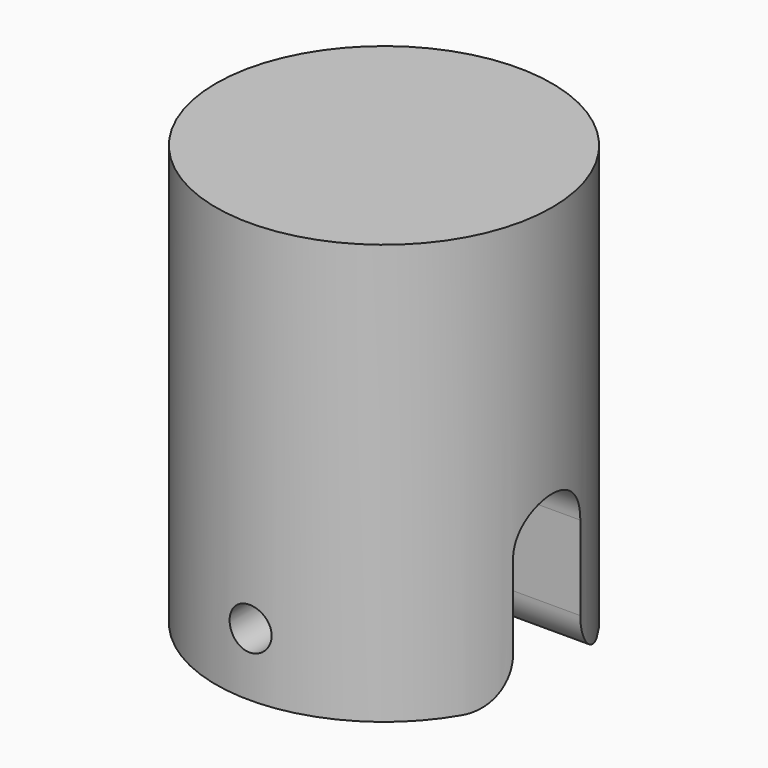
from build123d import *

# Parameters (mm, degrees)
F0_R     = 8
F1_DEPTH = 20
F3_DEPTH = 8
F5_D     = 2
F5_DEPTH = 6.001
F7_D     = 2
F8_R     = 2
F9_R     = 1.9999


# Not quite as in the source:
# - a fillet or chamfer is up to 0.001 mm smaller than in the source, because OpenCascade refuses the exact size


with BuildPart() as f1:
    # F0 (on Top) → F1 (new body)
    with BuildSketch(Plane.XY):
        Circle(F0_R)
    extrude(amount=F1_DEPTH)

    # F2 (on face) → F3 (cut)
    with BuildSketch(Plane.XY):
        with BuildLine():
            ThreePointArc((8, 0), (7.9362375701, 1.0080343399), (7.7459666924, 2))
            Line((7.7459666924, 2), (-7.7459666924, 2))
            ThreePointArc((-7.7459666924, 2), (-7.9362375701, 1.0080343399), (-8, 0))
            ThreePointArc((-8, 0), (-7.9362375701, -1.0080343399), (-7.7459666924, -2))
            Line((-7.7459666924, -2), (7.7459666924, -2))
            ThreePointArc((7.7459666924, -2), (7.9362375701, -1.0080343399), (8, 0))
        make_face()
    extrude(amount=F3_DEPTH, mode=Mode.SUBTRACT)

    # F5 (through all, one way)
    with BuildSketch(Plane(origin=(0, -2, 0), x_dir=(-1, 0, 0), z_dir=(0, 1, 0))):
        with Locations((0, 3)):
            Circle(F5_D / 2)
    extrude(amount=-F5_DEPTH, mode=Mode.SUBTRACT)

    # F7 (through all)
    with Locations(Plane.XZ.offset(-2)):
        with Locations((0, 3)):
            Hole(F7_D / 2)

    # F8
    f8_edges = [f1.edges().sort_by_distance(p)[0] for p in [
        (0, 2, 0),
        (0, -2, 0),
    ]]
    fillet(f8_edges, radius=F8_R)

    # F9 (radius 2 in the source; OpenCascade refuses exactly that, so slightly less here)
    f9_edges = [f1.edges().sort_by_distance(p)[0] for p in [
        (0, 2, 8),
        (0, -2, 8),
    ]]
    fillet(f9_edges, radius=F9_R)


solid = f1.part
